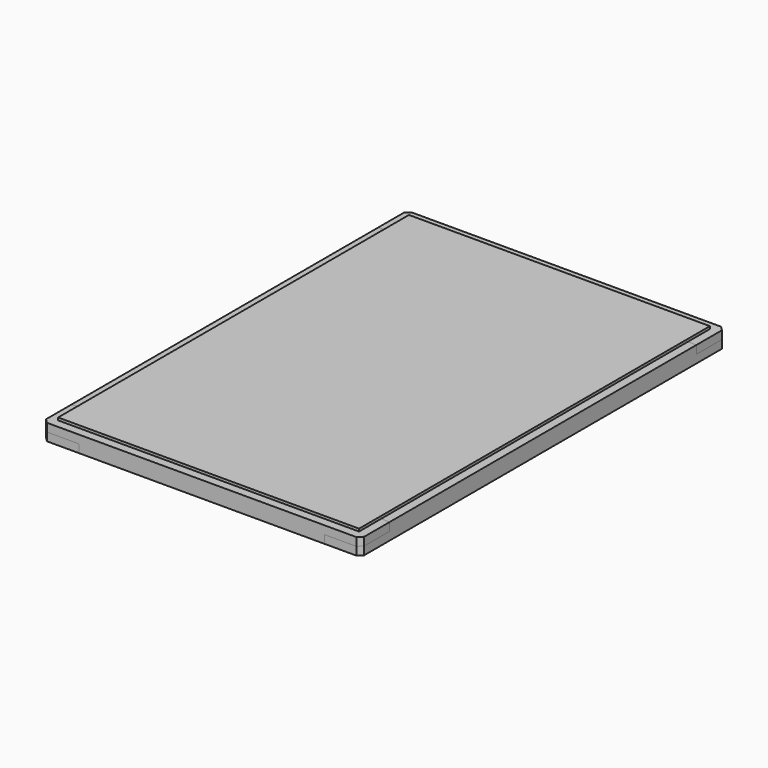
from build123d import *

# Parameters (mm, degrees)
F3_W      = 350
F3_H      = 510
F4_DEPTH  = 3
F5_W      = 350
F5_H      = 32
F5_R      = 4
F6_DEPTH  = 19
F7_W      = 42
F7_H      = 42
F7_R      = 4
F8_DEPTH  = 9.5
F9_SIZE   = 5
F11_W     = 32
F11_H     = 510
F11_R     = 4
F12_DEPTH = 19
F13_W     = 42
F13_H     = 42
F13_R     = 4
F14_DEPTH = 9.5
F15_SIZE  = 5
F17_R     = 4
F18_DEPTH = 19
F22_W     = 306
F22_H     = 466
F22_W_2   = 286
F22_H_2   = 446
F23_DEPTH = 10


# Not quite as in the source:
# - a feature names something its author has since deleted; it is built from what else it names


with BuildPart() as f4:
    # F3 (on Top) → F4 (new body)
    with BuildSketch(Plane.XY):
        Rectangle(F3_W, F3_H)
    extrude(amount=F4_DEPTH)


with BuildPart() as f6:
    # F5 (on face) → F6 (new body)
    with BuildSketch(Plane(origin=(0, 0, 0), x_dir=(1, 0, 0), z_dir=(0, 0, -1))):
        Polygon((-185, -265), (185, -265), (185, -223), (175, -223), (175, -255), (-175, -255), (-175, -223), (-185, -223), align=None)
        with Locations((0, -239)):
            Rectangle(F5_W, F5_H)
        with Locations((-164, -244)):
            Circle(F5_R, mode=Mode.SUBTRACT)
        with Locations((164, -244)):
            Circle(F5_R, mode=Mode.SUBTRACT)
    extrude(amount=F6_DEPTH)

    # F7 (on face) → F8 (cut)
    with BuildSketch(Plane(origin=(0, 0, -19), x_dir=(1, 0, 0), z_dir=(0, 0, -1))):
        with Locations((-164, -244)):
            Rectangle(F7_W, F7_H)
        with Locations((-164, -244)):
            Circle(F7_R, mode=Mode.SUBTRACT)
        with Locations((164, -244)):
            Rectangle(F7_W, F7_H)
        with Locations((164, -244)):
            Circle(F7_R, mode=Mode.SUBTRACT)
    extrude(amount=-F8_DEPTH, mode=Mode.SUBTRACT)

    # F9
    f9_edges = [f6.edges().sort_by_distance(p)[0] for p in [
        (-185, 265, -4.75),
        (185, 265, -4.75),
    ]]
    chamfer(f9_edges, length=F9_SIZE)


with BuildPart() as f10_1:
    # F10: instance of F6
    add(f6.part.mirror(Plane.XZ))


with BuildPart() as f12:
    # F11 (on face) → F12 (new body)
    with BuildSketch(Plane(origin=(0, 0, 0), x_dir=(1, 0, 0), z_dir=(0, 0, -1))):
        Polygon((-143, 265), (-185, 265), (-185, -265), (-143, -265), (-143, -255), (-175, -255), (-175, 255), (-143, 255), align=None)
        with Locations((-159, 0)):
            Rectangle(F11_W, F11_H)
        with Locations((-164, -244)):
            Circle(F11_R, mode=Mode.SUBTRACT)
        with Locations((-164, 244)):
            Circle(F11_R, mode=Mode.SUBTRACT)
    extrude(amount=F12_DEPTH)

    # F13 (on face) → F14 (cut)
    with BuildSketch(Plane.XY):
        with Locations((-164, 244)):
            Rectangle(F13_W, F13_H)
        with Locations((-164, 244)):
            Circle(F13_R, mode=Mode.SUBTRACT)
        with Locations((-164, -244)):
            Rectangle(F13_W, F13_H)
        with Locations((-164, -244)):
            Circle(F13_R, mode=Mode.SUBTRACT)
    extrude(amount=-F14_DEPTH, mode=Mode.SUBTRACT)

    # F15
    f15_edges = [f12.edges().sort_by_distance(p)[0] for p in [
        (-185, -265, -14.25),
        (-185, 265, -14.25),
    ]]
    chamfer(f15_edges, length=F15_SIZE)


with BuildPart() as f16_1:
    # F16: instance of F12
    add(f12.part.mirror(Plane.YZ))


with BuildPart() as f18:
    # F17 (on face) → F18 (new body)
    with BuildSketch(Plane(origin=(0, 0, 0), x_dir=(1, 0, 0), z_dir=(0, 0, -1))):
        with Locations((164, 244)):
            Circle(F17_R)
    extrude(amount=F18_DEPTH)


with BuildPart() as f19_1:
    # F19: instance of F18
    add(f18.part.mirror(Plane.YZ))


with BuildPart() as f20_1:
    # F20: instance of F18
    add(f18.part.mirror(Plane.XZ))


with BuildPart() as f20_2:
    # F20: instance of F19_1
    add(f19_1.part.mirror(Plane.XZ))


with BuildPart() as f23_tool:
    # F22 (on offset) → F23 (new body)
    with BuildSketch(Plane.XY.offset(-19)):
        Rectangle(F22_W, F22_H)
        Rectangle(F22_W_2, F22_H_2, mode=Mode.SUBTRACT)
    extrude(amount=F23_DEPTH)


with BuildPart() as f6_1:
    add(f6.part)

    # F23: cut by f23_tool
    add(f23_tool.part, mode=Mode.SUBTRACT)


with BuildPart() as f10_1_1:
    add(f10_1.part)

    # F23: cut by f23_tool
    add(f23_tool.part, mode=Mode.SUBTRACT)


with BuildPart() as f12_1:
    add(f12.part)

    # F23: cut by f23_tool
    add(f23_tool.part, mode=Mode.SUBTRACT)


with BuildPart() as f16_1_1:
    add(f16_1.part)

    # F23: cut by f23_tool
    add(f23_tool.part, mode=Mode.SUBTRACT)


solid = Compound([f4.part, f18.part, f19_1.part, f20_1.part, f20_2.part, f6_1.part, f10_1_1.part, f12_1.part, f16_1_1.part])
